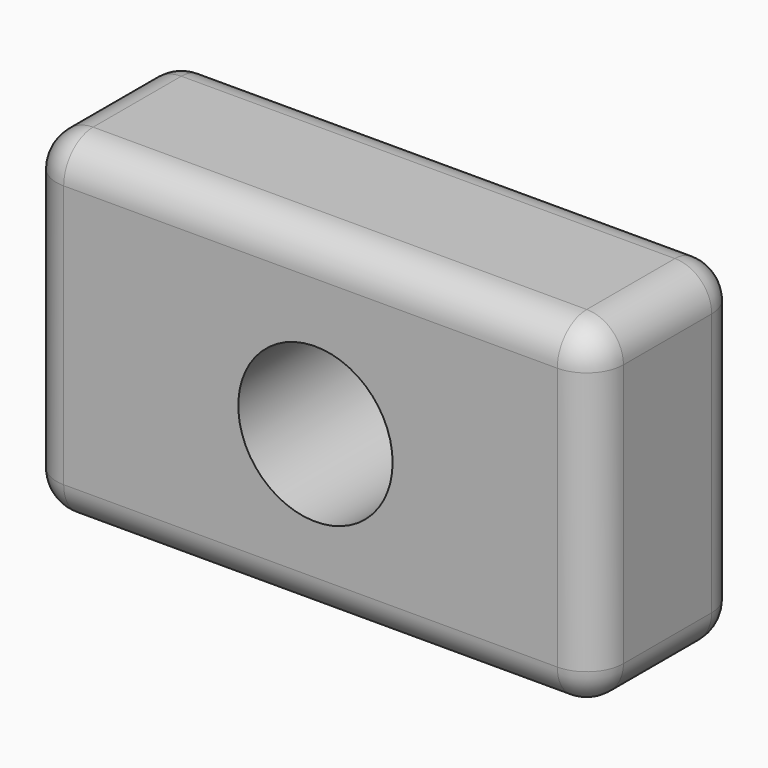
from build123d import *

# Parameters (mm, degrees)
F0_W         = 78.3818922937
F0_H         = 46.5174447745
F1_DEPTH     = 25.4
F2_R         = 5.08
F3_T1_DEPTH  = 15.24
F3_S5_W      = 5.08
F3_S5_H      = 5.08
F3_T6_DEPTH  = 5.08
F3_S11_W     = 5.08
F3_S11_H     = 5.08
F3_T12_DEPTH = 5.08
F4_R         = 10.6653295048
F5_DEPTH     = 25.4


# Not quite as in the source:
# - a fillet or chamfer that OpenCascade refuses, or shapes differently, is made with other operations: its cross-section is extruded or revolved along the edge and cut away or added


with BuildPart() as f1:
    # F0 (on Front) → F1 (new body)
    with BuildSketch(Plane.XZ):
        with Locations((1.8606986851, 2.9073404148)):
            Rectangle(F0_W, F0_H)
    extrude(amount=F1_DEPTH)

    # F2
    f2_edges = [f1.edges().sort_by_distance(p)[0] for p in [
        (41.051645, -12.7, 26.166063),
        (1.860699, -25.4, 26.166063),
        (1.860699, 0, 26.166063),
        (41.051645, -25.4, 2.90734),
        (41.051645, 0, 2.90734),
        (-37.330247, 0, 2.90734),
        (1.860699, 0, -20.351382),
        (41.051645, -12.7, -20.351382),
        (-37.330247, -12.7, -20.351382),
        (-37.330247, -25.4, 2.90734),
        (1.860699, -25.4, -20.351382),
    ]]
    fillet(f2_edges, radius=F2_R)

    # F3: fillet of radius 5.08 on 1 edges, made by hand

    # F3_s2 → F3_t1 (cut)
    with BuildSketch(Plane.XZ.offset(5.08)):
        with BuildLine():
            ThreePointArc((-32.2502474618, 26.1660628021), (-35.8423499102, 24.6781652505), (-37.3302474618, 21.0860628021))
            Line((-37.3302474618, 21.0860628021), (-37.3302474618, 26.1660628021))
            Line((-37.3302474618, 26.1660628021), (-32.2502474618, 26.1660628021))
        make_face()
    extrude(amount=F3_T1_DEPTH, mode=Mode.SUBTRACT)


with BuildPart() as f3_tool4:
    # F3_s5 → F3_t6 (new body)
    with BuildSketch(Plane.XY.offset(21.0860628021)):
        with Locations((-34.7902474618, -2.54)):
            Rectangle(F3_S5_W, F3_S5_H)
    extrude(amount=F3_T6_DEPTH)

    # F3_s7 → F3_t8 (revolve, cut)
    with BuildSketch(Plane(origin=(-32.2502474618, -5.08, 21.0860628021), x_dir=(0.7071067812, -0.7071067812, 0), z_dir=(-0.7071067812, -0.7071067812, 0))):
        with BuildLine():
            ThreePointArc((0, -5.08), (5.08, 0), (0, 5.08))
            Line((0, 5.08), (0, -5.08))
        make_face()
    revolve(axis=Axis((-32.2502474618, -5.08, 21.0860628021), (0, 0, 1)), mode=Mode.SUBTRACT)


with BuildPart() as f1_1:
    add(f1.part)

    # F3_t3: cut F3_tool4
    add(f3_tool4.part, mode=Mode.SUBTRACT)


with BuildPart() as f3_tool10:
    # F3_s11 → F3_t12 (new body)
    with BuildSketch(Plane.XY.offset(21.0860628021)):
        with Locations((-34.7902474618, -22.86)):
            Rectangle(F3_S11_W, F3_S11_H)
    extrude(amount=F3_T12_DEPTH)

    # F3_s13 → F3_t14 (revolve, cut)
    with BuildSketch(Plane(origin=(-32.2502474618, -20.32, 21.0860628021), x_dir=(0.7071067812, 0.7071067812, 0), z_dir=(0.7071067812, -0.7071067812, 0))):
        with BuildLine():
            ThreePointArc((0, -5.08), (5.08, 0), (0, 5.08))
            Line((0, 5.08), (0, -5.08))
        make_face()
    revolve(axis=Axis((-32.2502474618, -20.32, 21.0860628021), (0, 0, 1)), mode=Mode.SUBTRACT)


with BuildPart() as f1_2:
    add(f1_1.part)

    # F3_t9: cut F3_tool10
    add(f3_tool10.part, mode=Mode.SUBTRACT)

    # F4 (on face) → F5 (cut, through all)
    with BuildSketch(Plane.XZ.offset(25.4)):
        with Locations((2.5458505843, 2.2031988483)):
            Circle(F4_R)
    extrude(amount=-F5_DEPTH, mode=Mode.SUBTRACT)


solid = f1_2.part
